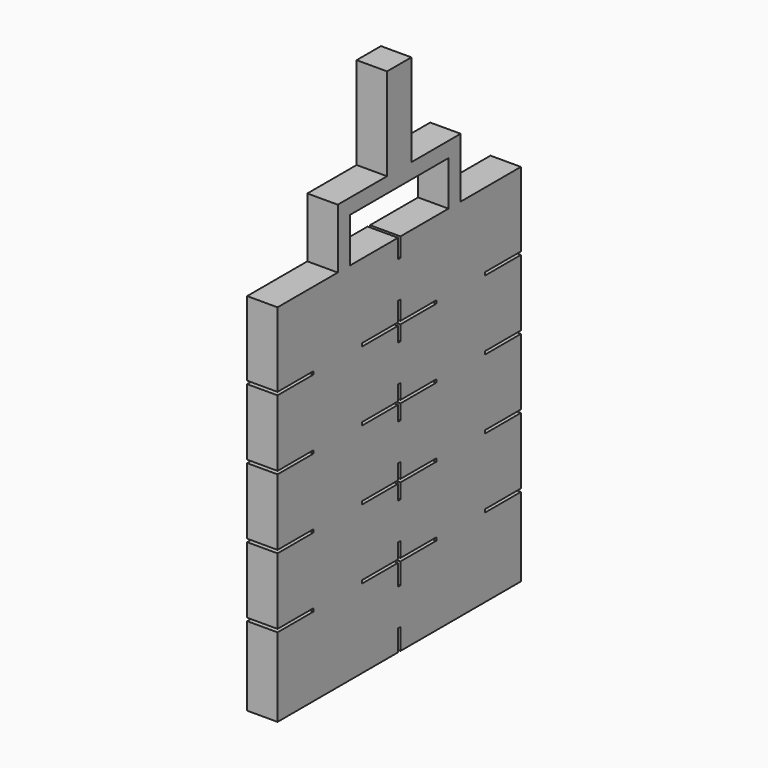
from build123d import *

# Parameters (mm, degrees)
F1_DEPTH = 5


# Not quite as in the source:
# - a feature names something its author has since deleted; it is built from what else it names


with BuildPart() as f1:
    # F0 (on Right) → F1 (new body)
    with BuildSketch(Plane.YZ):
        Polygon((12.375, 0), (0, 0), (0, -12.238), (7.3750000447, -12.238), (7.3750000447, -12.738), (0, -12.738), (0, -23.672), (7.3750000447, -23.672), (7.3750000447, -24.172), (0, -24.172), (0, -35.106), (7.3750000447, -35.106), (7.3750000447, -35.606), (0, -35.606), (0, -46.54), (7.3750000447, -46.54), (7.3750000447, -47.04), (0, -47.04), (0, -60), (24.75, -60), (24.75, -56.52), (25.25, -56.52), (25.25, -60), (50, -60), (50, -47.04), (42.6249988377, -47.04), (42.6249988377, -46.54), (50, -46.54), (50, -35.606), (42.6249988377, -35.606), (42.6249988377, -35.106), (50, -35.106), (50, -24.172), (42.6249988377, -24.172), (42.6249988377, -23.672), (50, -23.672), (50, -12.738), (42.6249988377, -12.738), (42.6249988377, -12.238), (50, -12.238), (50, 0), (37.625, 0), (37.625, 9.8238829523), (27.5, 9.8238829523), (27.5, 25), (22.5, 25), (22.5, 9.8238829523), (12.375, 9.8238829523), align=None)
        Polygon((25.25, -44.073), (25.25, -46.54), (32.625, -46.54), (32.625, -47.04), (25.25, -47.04), (25.25, -50.52), (24.75, -50.52), (24.75, -47.04), (17.375, -47.04), (17.375, -46.54), (24.75, -46.54), (24.75, -44.073), align=None, mode=Mode.SUBTRACT)
        Polygon((25.25, -32.639), (25.25, -35.106), (32.625, -35.106), (32.625, -35.606), (25.25, -35.606), (25.25, -38.073), (24.75, -38.073), (24.75, -35.606), (17.375, -35.606), (17.375, -35.106), (24.75, -35.106), (24.75, -32.639), align=None, mode=Mode.SUBTRACT)
        Polygon((25.25, -21.205), (25.25, -23.672), (32.625, -23.672), (32.625, -24.172), (25.25, -24.172), (25.25, -26.639), (24.75, -26.639), (24.75, -24.172), (17.375, -24.172), (17.375, -23.672), (24.75, -23.672), (24.75, -21.205), align=None, mode=Mode.SUBTRACT)
        Polygon((25.25, -9.119), (25.25, -12.238), (32.625, -12.238), (32.625, -12.738), (25.25, -12.738), (25.25, -15.205), (24.75, -15.205), (24.75, -12.738), (17.375, -12.738), (17.375, -12.238), (24.75, -12.238), (24.75, -9.119), align=None, mode=Mode.SUBTRACT)
        Polygon((25.25, -1.304), (25.25, -3.119), (24.75, -3.119), (24.75, 0), (14.875, 0), (14.875, 7.3238829523), (35.125, 7.3238829523), (35.125, 0), (25.25, 0), align=None, mode=Mode.SUBTRACT)
    extrude(amount=F1_DEPTH)


solid = f1.part
